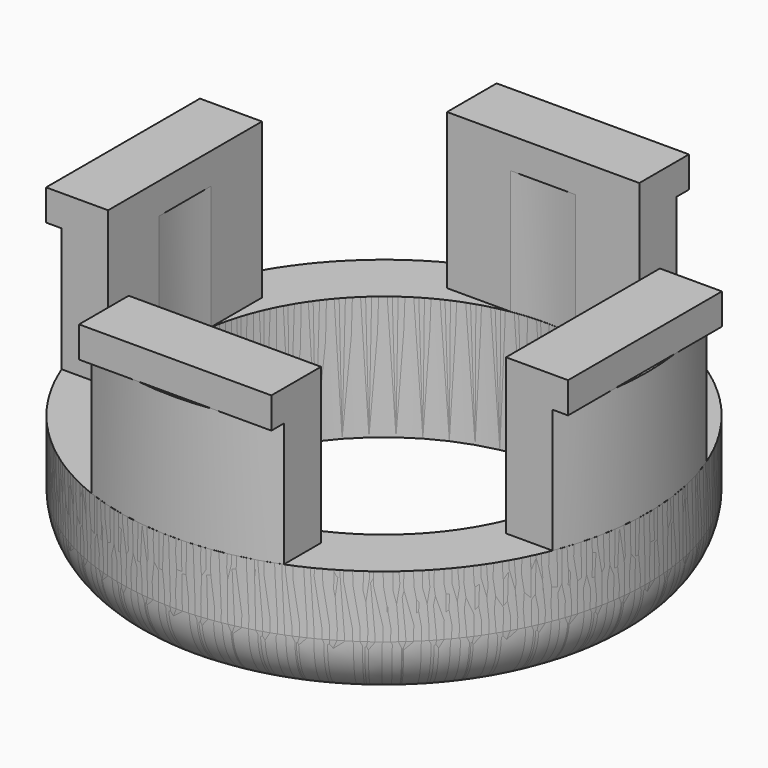
from build123d import *

# Parameters (mm, degrees)
F0_R     = 8.5
F0_R_2   = 6.5
F1_DEPTH = 4
F2_R     = 1.99999
F4_DEPTH = 4
F5_W     = 6.2004313804
F5_H     = 2
F6_DEPTH = 1
F8_COUNT = 4


# Not quite as in the source:
# - a fillet or chamfer is up to 0.001 mm smaller than in the source, because OpenCascade refuses the exact size


with BuildPart() as f1:
    # F0 (on Top) → F1 (new body)
    with BuildSketch(Plane.XY):
        Circle(F0_R)
        Circle(F0_R_2, mode=Mode.SUBTRACT)
    extrude(amount=F1_DEPTH)

    # F2 (radius 2 in the source; OpenCascade refuses exactly that, so slightly less here)
    f2_edges = [f1.edges().sort_by_distance(p)[0] for p in [
        (-8.5, 0, 0),
    ]]
    fillet(f2_edges, radius=F2_R)

    # F3 (on face) → F4 (join)
    with BuildSketch(Plane.XY.offset(4)):
        with BuildLine():
            Line((-1.0496680978, -6.4146860316), (-3.1002156902, -6.4146860316))
            Line((-3.1002156902, -6.4146860316), (-3.1002156902, -7.9144590892))
            ThreePointArc((-3.1002156902, -7.9144590892), (0, -8.5), (3.1002156902, -7.9144590892))
            Line((3.1002156902, -7.9144590892), (3.1002156902, -6.4146860316))
            Line((3.1002156902, -6.4146860316), (1.0496680978, -6.4146860316))
            ThreePointArc((1.0496680978, -6.4146860316), (0, -6.5), (-1.0496680978, -6.4146860316))
        make_face()
    extrude(amount=F4_DEPTH)

    # F5 (on face) → F6 (join)
    with BuildSketch(Plane.XY.offset(8)):
        with Locations((0, -7.4146860316)):
            Rectangle(F5_W, F5_H)
    extrude(amount=F6_DEPTH)


with BuildPart() as f8_1:
    # F8: instance of F1
    add(f1.part.rotate(Axis((0, 0, 10.2825174108), (0, 0, 1)), 1 * 360 / F8_COUNT))


with BuildPart() as f8_2:
    # F8: instance of F1
    add(f1.part.rotate(Axis((0, 0, 10.2825174108), (0, 0, 1)), 2 * 360 / F8_COUNT))


with BuildPart() as f8_3:
    # F8: instance of F1
    add(f1.part.rotate(Axis((0, 0, 10.2825174108), (0, 0, 1)), 3 * 360 / F8_COUNT))


solid = Compound([f1.part, f8_1.part, f8_2.part, f8_3.part])
